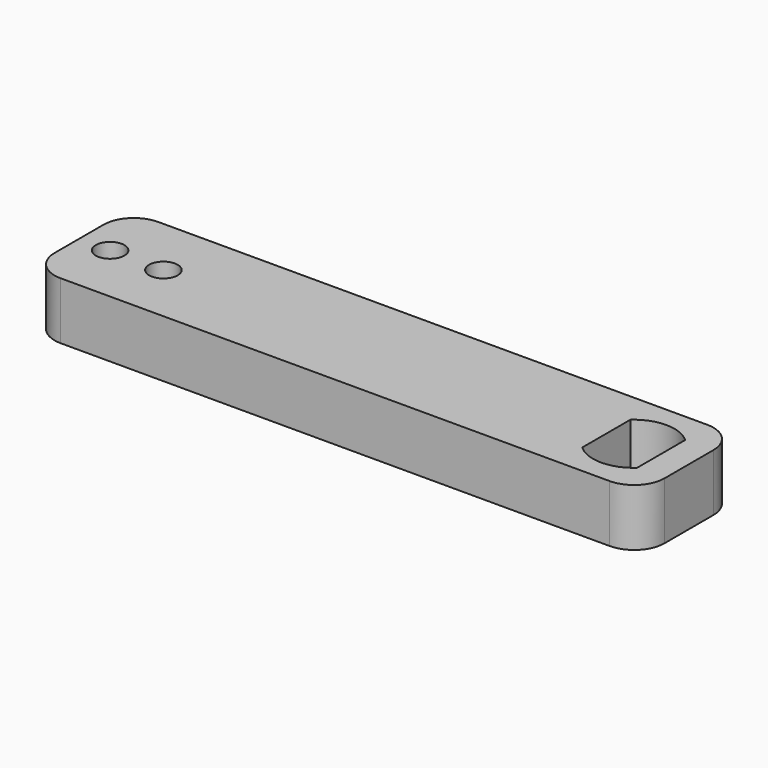
from build123d import *

# Parameters (mm, degrees)
F1_DEPTH = 4.7625
F2_R     = 2.54


# Not quite as in the source:
# - a length typed as a fraction of an inch, garbled in the dataset ("3 / 203.2 mm" for 3/8 in), is restored


with BuildPart() as f1:
    # F0 (on Top) → F1 (new body)
    with BuildSketch(Plane.XY):
        with BuildLine():
            Line((23.4723398992, 10.7888607308), (23.4723398992, 15.8688607308))
            Line((23.4723398992, 15.8688607308), (-27.3276601008, 15.8688607308))
            Line((-27.3276601008, 15.8688607308), (-27.3276601008, 10.7888607308))
            Line((-27.3276601008, 10.7888607308), (-25.9275856725, 10.7888607308))
            ThreePointArc((-25.9275856725, 10.7888607308), (-24.7369606725, 11.9794857308), (-23.5463356725, 10.7888607308))
            Line((-23.5463356725, 10.7888607308), (-21.4888538531, 10.7888607308))
            ThreePointArc((-21.4888538531, 10.7888607308), (-20.2982288531, 11.9794857308), (-19.1076038531, 10.7888607308))
            Line((-19.1076038531, 10.7888607308), (15.4761500436, 10.7888607308))
            ThreePointArc((15.4761500436, 10.7888607308), (15.7646477316, 12.1575472198), (16.5810500436, 13.2933380835))
            ThreePointArc((16.5810500436, 13.2933380835), (18.8670500436, 14.1797607308), (21.1530500436, 13.2933380835))
            ThreePointArc((21.1530500436, 13.2933380835), (21.9694523555, 12.1575472198), (22.2579500436, 10.7888607308))
            Line((22.2579500436, 10.7888607308), (23.4723398992, 10.7888607308))
        make_face()
        with BuildLine():
            Line((23.4723398992, 5.7088607308), (23.4723398992, 10.7888607308))
            Line((23.4723398992, 10.7888607308), (22.2579500436, 10.7888607308))
            ThreePointArc((22.2579500436, 10.7888607308), (21.9694523555, 9.4201742419), (21.1530500436, 8.2843833782))
            ThreePointArc((21.1530500436, 8.2843833782), (18.8670500436, 7.3979607308), (16.5810500436, 8.2843833782))
            ThreePointArc((16.5810500436, 8.2843833782), (15.7646477316, 9.4201742419), (15.4761500436, 10.7888607308))
            Line((15.4761500436, 10.7888607308), (-19.1076038531, 10.7888607308))
            ThreePointArc((-19.1076038531, 10.7888607308), (-20.2982288531, 9.5982357308), (-21.4888538531, 10.7888607308))
            Line((-21.4888538531, 10.7888607308), (-23.5463356725, 10.7888607308))
            ThreePointArc((-23.5463356725, 10.7888607308), (-24.7369606725, 9.5982357308), (-25.9275856725, 10.7888607308))
            Line((-25.9275856725, 10.7888607308), (-27.3276601008, 10.7888607308))
            Line((-27.3276601008, 10.7888607308), (-27.3276601008, 5.7088607308))
            Line((-27.3276601008, 5.7088607308), (23.4723398992, 5.7088607308))
        make_face()
        with BuildLine():
            Line((16.5810500436, 8.2843833782), (16.5810500436, 10.7888607308))
            Line((16.5810500436, 10.7888607308), (15.4761500436, 10.7888607308))
            ThreePointArc((15.4761500436, 10.7888607308), (15.7646477316, 9.4201742419), (16.5810500436, 8.2843833782))
        make_face()
        with BuildLine():
            Line((15.4761500436, 10.7888607308), (16.5810500436, 10.7888607308))
            Line((16.5810500436, 10.7888607308), (16.5810500436, 13.2933380835))
            ThreePointArc((16.5810500436, 13.2933380835), (15.7646477316, 12.1575472198), (15.4761500436, 10.7888607308))
        make_face()
        with BuildLine():
            Line((21.1530500436, 10.7888607308), (22.2579500436, 10.7888607308))
            ThreePointArc((22.2579500436, 10.7888607308), (21.9694523555, 12.1575472198), (21.1530500436, 13.2933380835))
            Line((21.1530500436, 13.2933380835), (21.1530500436, 10.7888607308))
        make_face()
        with BuildLine():
            ThreePointArc((21.1530500436, 8.2843833782), (21.9694523555, 9.4201742419), (22.2579500436, 10.7888607308))
            Line((22.2579500436, 10.7888607308), (21.1530500436, 10.7888607308))
            Line((21.1530500436, 10.7888607308), (21.1530500436, 8.2843833782))
        make_face()
    extrude(amount=F1_DEPTH)

    # F2
    f2_edges = [f1.edges().sort_by_distance(p)[0] for p in [
        (23.47234, 15.868861, 2.38125),
        (-27.32766, 15.868861, 2.38125),
        (-27.32766, 5.708861, 2.38125),
        (23.47234, 5.708861, 2.38125),
    ]]
    fillet(f2_edges, radius=F2_R)


solid = f1.part
